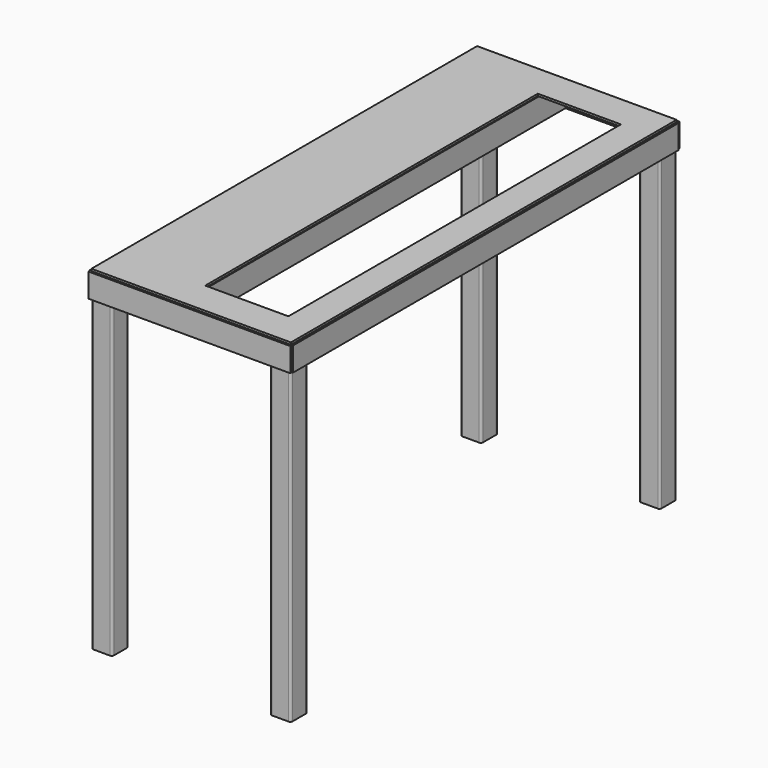
from build123d import *

# Parameters (mm, degrees)
F0_W      = 304.8
F0_H      = 736.6
F0_W_2    = 127
F0_H_2    = 635
F1_DEPTH  = 3.175
F2_W      = 736.6
F2_H      = 36.5125
F3_DEPTH  = 3.175
F5_W      = 307.975
F5_H      = 36.5125
F6_DEPTH  = 3.175
F9_W      = 736.6
F9_H      = 36.5125
F10_DEPTH = 1.5875
F13_DEPTH = 1.5875
F15_W     = 123.825
F15_H     = 36.5125
F16_DEPTH = 1.5875
F17_W     = 26.67
F17_H     = 26.67
F18_DEPTH = 508


with BuildPart() as f1:
    # F0 (on Top) → F1 (new body)
    with BuildSketch(Plane.XY):
        Rectangle(F0_W, F0_H)
        with Locations((44.45, 0)):
            Rectangle(F0_W_2, F0_H_2, mode=Mode.SUBTRACT)
    extrude(amount=F1_DEPTH)


with BuildPart() as f3:
    # F2 (on face) → F3 (new body)
    with BuildSketch(Plane.YZ.offset(152.4)):
        with Locations((0, -18.25625)):
            Rectangle(F2_W, F2_H)
    extrude(amount=F3_DEPTH)


with BuildPart() as f4_1:
    # F4: instance of F3
    add(f3.part.mirror(Plane.YZ))


with BuildPart() as f6:
    # F5 (on face) → F6 (new body)
    with BuildSketch(Plane.XZ.offset(368.3)):
        with Locations((0, -18.25625)):
            Rectangle(F5_W, F5_H)
    extrude(amount=F6_DEPTH)


with BuildPart() as f7_1:
    # F7: instance of F6
    add(f6.part.mirror(Plane.XZ))


with BuildPart() as f10:
    # F9 (on face) → F10 (new body, symmetric)
    with BuildSketch(Plane(origin=(-19.05, 0, 0), x_dir=(0, -1, 0), z_dir=(-1, 0, 0))):
        with Locations((0, -18.25625)):
            Rectangle(F9_W, F9_H)
    extrude(amount=F10_DEPTH, both=True)


with BuildPart() as f13:
    # F12 (on face) → F13 (new body, symmetric)
    with BuildSketch(Plane.YZ.offset(107.95)):
        Polygon((368.3, 0), (317.5, 0), (-317.5, 0), (-368.3, 0), (-368.3, -36.5125), (368.3, -36.5125), align=None)
    extrude(amount=F13_DEPTH, both=True)


with BuildPart() as f16:
    # F15 (on face) → F16 (new body, symmetric)
    with BuildSketch(Plane(origin=(0, -317.5, 0), x_dir=(-1, 0, 0), z_dir=(0, 1, 0))):
        with Locations((-44.45, -18.25625)):
            Rectangle(F15_W, F15_H)
    extrude(amount=F16_DEPTH, both=True)


with BuildPart() as f18:
    # F17 (on face) → F18 (new body)
    with BuildSketch(Plane(origin=(0, 0, 0), x_dir=(1, 0, 0), z_dir=(0, 0, -1))):
        with BuildLine():
            Line((-123.825, 368.3), (-149.225, 368.3))
            ThreePointArc((-149.225, 368.3), (-151.4700640303, 367.3700640303), (-152.4, 365.125))
            Line((-152.4, 365.125), (-152.4, 339.725))
            ThreePointArc((-152.4, 339.725), (-151.4700640303, 337.4799359697), (-149.225, 336.55))
            Line((-149.225, 336.55), (-123.825, 336.55))
            ThreePointArc((-123.825, 336.55), (-121.5799359697, 337.4799359697), (-120.65, 339.725))
            Line((-120.65, 339.725), (-120.65, 365.125))
            ThreePointArc((-120.65, 365.125), (-121.5799359697, 367.3700640303), (-123.825, 368.3))
        make_face()
        with Locations((-136.525, 352.425)):
            Rectangle(F17_W, F17_H, mode=Mode.SUBTRACT)
    extrude(amount=F18_DEPTH)


with BuildPart() as f18b:
    # F17 (on face) → F18, piece 2 (new body)
    with BuildSketch(Plane(origin=(0, 0, 0), x_dir=(1, 0, 0), z_dir=(0, 0, -1))):
        with BuildLine():
            Line((-120.65, -365.125), (-120.65, -339.725))
            ThreePointArc((-120.65, -339.725), (-121.5799359697, -337.4799359697), (-123.825, -336.55))
            Line((-123.825, -336.55), (-149.225, -336.55))
            ThreePointArc((-149.225, -336.55), (-151.4700640303, -337.4799359697), (-152.4, -339.725))
            Line((-152.4, -339.725), (-152.4, -365.125))
            ThreePointArc((-152.4, -365.125), (-151.4700640303, -367.3700640303), (-149.225, -368.3))
            Line((-149.225, -368.3), (-123.825, -368.3))
            ThreePointArc((-123.825, -368.3), (-121.5799359697, -367.3700640303), (-120.65, -365.125))
        make_face()
        with Locations((-136.525, -352.425)):
            Rectangle(F17_W, F17_H, mode=Mode.SUBTRACT)
    extrude(amount=F18_DEPTH)


with BuildPart() as f18c:
    # F17 (on face) → F18, piece 3 (new body)
    with BuildSketch(Plane(origin=(0, 0, 0), x_dir=(1, 0, 0), z_dir=(0, 0, -1))):
        with BuildLine():
            Line((152.2095, 339.725), (152.2095, 365.125))
            ThreePointArc((152.2095, 365.125), (151.2795640303, 367.3700640303), (149.0345, 368.3))
            Line((149.0345, 368.3), (123.6345, 368.3))
            ThreePointArc((123.6345, 368.3), (121.3894359697, 367.3700640303), (120.4595, 365.125))
            Line((120.4595, 365.125), (120.4595, 339.725))
            ThreePointArc((120.4595, 339.725), (121.3894359697, 337.4799359697), (123.6345, 336.55))
            Line((123.6345, 336.55), (149.0345, 336.55))
            ThreePointArc((149.0345, 336.55), (151.2795640303, 337.4799359697), (152.2095, 339.725))
        make_face()
        with Locations((136.3345, 352.425)):
            Rectangle(F17_W, F17_H, mode=Mode.SUBTRACT)
    extrude(amount=F18_DEPTH)


with BuildPart() as f18d:
    # F17 (on face) → F18, piece 4 (new body)
    with BuildSketch(Plane(origin=(0, 0, 0), x_dir=(1, 0, 0), z_dir=(0, 0, -1))):
        with BuildLine():
            Line((152.2095, -365.125), (152.2095, -339.725))
            ThreePointArc((152.2095, -339.725), (151.2795640303, -337.4799359697), (149.0345, -336.55))
            Line((149.0345, -336.55), (123.6345, -336.55))
            ThreePointArc((123.6345, -336.55), (121.3894359697, -337.4799359697), (120.4595, -339.725))
            Line((120.4595, -339.725), (120.4595, -365.125))
            ThreePointArc((120.4595, -365.125), (121.3894359697, -367.3700640303), (123.6345, -368.3))
            Line((123.6345, -368.3), (149.0345, -368.3))
            ThreePointArc((149.0345, -368.3), (151.2795640303, -367.3700640303), (152.2095, -365.125))
        make_face()
        with Locations((136.3345, -352.425)):
            Rectangle(F17_W, F17_H, mode=Mode.SUBTRACT)
    extrude(amount=F18_DEPTH)


solid = Compound([f1.part, f3.part, f4_1.part, f6.part, f7_1.part, f10.part, f13.part, f16.part, f18.part, f18b.part, f18c.part, f18d.part])
